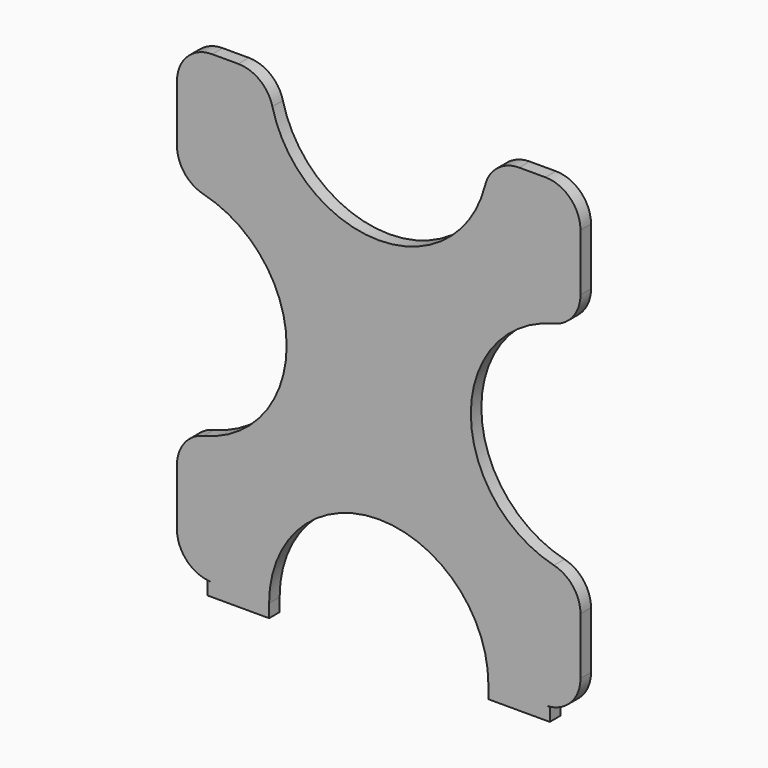
from build123d import *

# Parameters (mm, degrees)
F2_DEPTH = 19.05
F3_R     = 50.8
F4_W     = 88.9
F4_H     = 19.05
F5_DEPTH = 19.05


# Not quite as in the source:
# - a variable given as a bare number and used for a length is read in inches; the dataset says mm whatever the document's units were


with BuildPart() as f2:
    # F1 (on Front) → F2 (new body)
    with BuildSketch(Plane.XZ):
        with BuildLine():
            Line((292.1, 336.55), (158.75, 336.55))
            ThreePointArc((158.75, 336.55), (0, 177.8), (-158.75, 336.55))
            Line((-158.75, 336.55), (-292.1, 336.55))
            Line((-292.1, 336.55), (-292.1, 158.75))
            ThreePointArc((-292.1, 158.75), (-179.8467984866, 112.2532015134), (-133.35, 0))
            ThreePointArc((-133.35, 0), (-179.8467984866, -112.2532015134), (-292.1, -158.75))
            Line((-292.1, -158.75), (-292.1, -336.55))
            Line((-292.1, -336.55), (-158.75, -336.55))
            ThreePointArc((-158.75, -336.55), (0, -177.8), (158.75, -336.55))
            Line((158.75, -336.55), (292.1, -336.55))
            Line((292.1, -336.55), (292.1, -158.75))
            ThreePointArc((292.1, -158.75), (133.35, 0), (292.1, 158.75))
            Line((292.1, 158.75), (292.1, 336.55))
        make_face()
    extrude(amount=F2_DEPTH)

    # F3
    f3_edges = [f2.edges().sort_by_distance(p)[0] for p in [
        (158.75, -9.525, 336.55),
        (-158.75, -9.525, 336.55),
        (292.1, -9.525, 158.75),
        (292.1, -9.525, -158.75),
        (-292.1, -9.525, -158.75),
        (-292.1, -9.525, 158.75),
        (292.1, -9.525, -336.55),
        (-292.1, -9.525, -336.55),
        (292.1, -9.525, 336.55),
        (-292.1, -9.525, 336.55),
    ]]
    fillet(f3_edges, radius=F3_R)

    # F4 (on face) → F5 (join)
    with BuildSketch(Plane(origin=(0, 0, -336.55), x_dir=(1, 0, 0), z_dir=(0, 0, -1))):
        with Locations((-203.2, 9.525)):
            Rectangle(F4_W, F4_H)
        with Locations((203.2, 9.525)):
            Rectangle(F4_W, F4_H)
    extrude(amount=F5_DEPTH)


solid = f2.part
